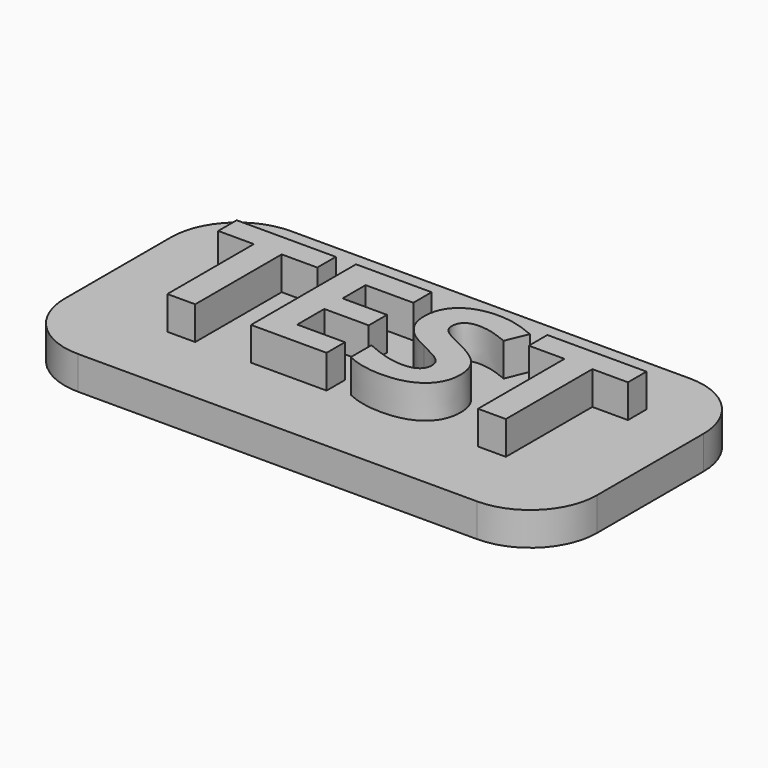
from build123d import *

# Parameters (mm, degrees)
F0_W         = 12.7
F0_H         = 6.35
F1_DEPTH     = 0.79375
F2_R         = 1.5875
F3_TEXT_SIZE = 4.386512996
F4_DEPTH     = 0.79375


# Not quite as in the source:
# - Text() gives the source's letters only with a copy of the font that has no kerning and outlines rounded to 1/6400 em; it was checked with that copy


with BuildPart() as f1:
    # F0 (on Top) → F1 (new body)
    with BuildSketch(Plane.XY):
        Rectangle(F0_W, F0_H)
    extrude(amount=F1_DEPTH)

    # F2
    f2_edges = [f1.edges().sort_by_distance(p)[0] for p in [
        (-6.35, -3.175, 0.396875),
        (6.35, 3.175, 0.396875),
        (6.35, -3.175, 0.396875),
        (-6.35, 3.175, 0.396875),
    ]]
    fillet(f2_edges, radius=F2_R)

    # F3 (on face) → F4 (join)
    with BuildSketch(Plane.XY.offset(0.79375)):
        with Locations((-4.9583842465, -1.436176839)):
            Text('TEST', F3_TEXT_SIZE, font='Open Sans', font_style=FontStyle.BOLD, text_align=(TextAlign.LEFT, TextAlign.BOTTOM))
    extrude(amount=F4_DEPTH)


solid = f1.part
